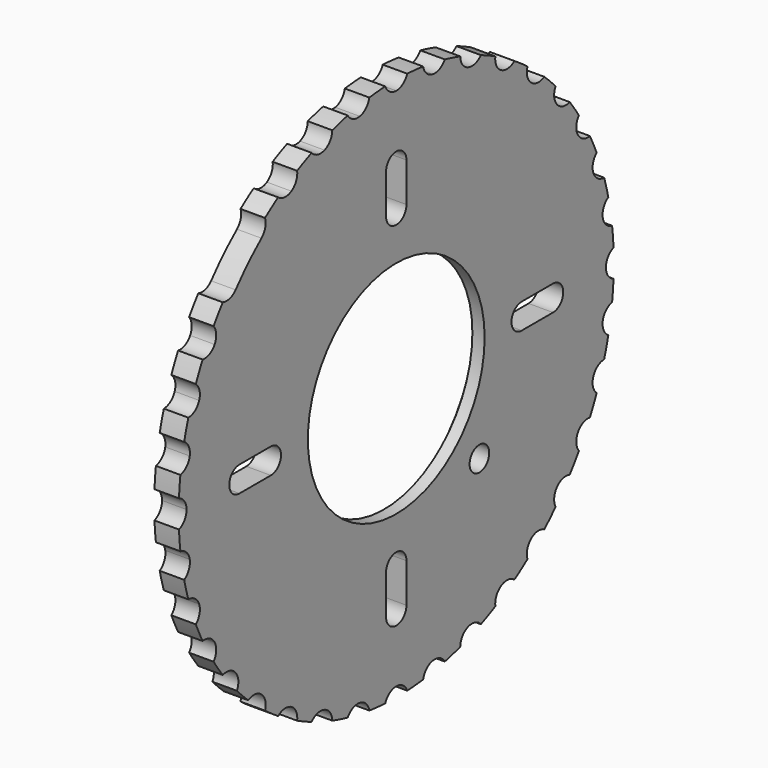
from build123d import *

# Parameters (mm, degrees)
F0_R     = 2.5
F0_R_2   = 26.25
F2_DEPTH = 5
F1_START = 2.5
F0_R_3   = 22.55
F1_DEPTH = 2.5


# Not quite as in the source:
# - a feature names something its author has since deleted; it is built from what else it names


with BuildPart() as f2:
    # F0 (on Right) → F2 (new body)
    with BuildSketch(Plane.YZ):
        with BuildLine():
            ThreePointArc((0, 53.5), (4.6628322594, 53.296416346), (9.2901775494, 52.6872147784))
            ThreePointArc((9.2901775494, 52.6872147784), (7.7067499567, 53.5035037785), (6.8653638665, 55.0737394679))
            ThreePointArc((6.8653638665, 55.0737394679), (4.8371437225, 55.2888057441), (2.8023909329, 55.4292035398))
            ThreePointArc((2.8023909329, 55.4292035398), (1.7011188406, 54.0289284328), (0, 53.5))
        make_face()
        with BuildLine():
            ThreePointArc((9.2901775494, 52.6872147784), (13.8468189413, 51.6770316989), (18.2980776808, 50.2735552073))
            ThreePointArc((18.2980776808, 50.2735552073), (16.8804530287, 51.3524022613), (16.3245180589, 53.0448876909))
            ThreePointArc((16.3245180589, 53.0448876909), (14.3644570032, 53.608883359), (12.3849965019, 54.1004793107))
            ThreePointArc((12.3849965019, 54.1004793107), (11.0573000071, 52.9127114302), (9.2901775494, 52.6872147784))
        make_face()
        with BuildLine():
            ThreePointArc((18.2980776808, 50.2735552073), (22.6100768811, 48.4874666634), (26.7499997548, 46.332359244))
            ThreePointArc((26.7499997548, 46.332359244), (25.5412520248, 47.6409841102), (25.2876600307, 49.4042938435))
            ThreePointArc((25.2876600307, 49.4042938435), (23.4553135266, 50.3000821805), (21.5912902193, 51.1279393939))
            ThreePointArc((21.5912902193, 51.1279393939), (20.0775106745, 50.1887684493), (18.2980776808, 50.2735552073))
        make_face()
        with BuildLine():
            ThreePointArc((26.7499997548, 46.332359244), (30.6863392453, 43.8246344391), (34.3891371491, 40.983377681))
            ThreePointArc((34.3891371491, 40.983377681), (33.4259931317, 42.4820184875), (33.4824492486, 44.2625755274))
            ThreePointArc((33.4824492486, 44.2625755274), (31.8334922175, 45.462938458), (30.1415435091, 46.6019029106))
            ThreePointArc((30.1415435091, 46.6019029106), (28.4876762061, 45.9398651305), (26.7499997548, 46.332359244))
        make_face()
        with BuildLine():
            ThreePointArc((34.3891371491, 40.983377681), (37.8302128361, 37.8302127508), (40.9833777585, 34.3891370567))
            ThreePointArc((40.9833777585, 34.3891370567), (40.2951022841, 36.0322583562), (40.659891189, 37.7759612518))
            ThreePointArc((40.659891189, 37.7759612518), (39.2444263559, 39.2444263559), (37.7759612518, 40.659891189))
            ThreePointArc((37.7759612518, 40.659891189), (36.0322584162, 40.2951022784), (34.3891371491, 40.983377681))
        make_face()
        with BuildLine():
            ThreePointArc((40.9833777585, 34.3891370567), (43.8246344309, 30.686339257), (46.3323591695, 26.7499998839))
            ThreePointArc((46.3323591695, 26.7499998839), (45.9398651365, 28.4876762804), (46.6019029106, 30.1415435091))
            ThreePointArc((46.6019029106, 30.1415435091), (45.462938458, 31.8334922175), (44.2625755274, 33.4824492486))
            ThreePointArc((44.2625755274, 33.4824492486), (42.4820185456, 33.4259931156), (40.9833777585, 34.3891370567))
        make_face()
        with BuildLine():
            ThreePointArc((46.3323591695, 26.7499998839), (48.4874666685, 22.6100768701), (50.2735552666, 18.298077518))
            ThreePointArc((50.2735552666, 18.298077518), (50.1887684276, 20.0775105907), (51.1279393939, 21.5912902193))
            ThreePointArc((51.1279393939, 21.5912902193), (50.3000821805, 23.4553135266), (49.4042938435, 25.2876600307))
            ThreePointArc((49.4042938435, 25.2876600307), (47.6409840429, 25.5412520568), (46.3323591695, 26.7499998839))
        make_face()
        with BuildLine():
            ThreePointArc((50.2735552666, 18.298077518), (51.6770317213, 13.8468188576), (52.6872147784, 9.2901775494))
            ThreePointArc((52.6872147784, 9.2901775494), (52.9127114302, 11.0573000071), (54.1004793107, 12.3849965019))
            ThreePointArc((54.1004793107, 12.3849965019), (53.608883359, 14.3644570032), (53.0448876909, 16.3245180589))
            ThreePointArc((53.0448876909, 16.3245180589), (51.3524023319, 16.8804529785), (50.2735552666, 18.298077518))
        make_face()
        with BuildLine():
            ThreePointArc((52.6872147784, 9.2901775494), (53.296416346, 4.6628322594), (53.5, 0))
            ThreePointArc((53.5, 0), (54.0289284328, 1.7011188406), (55.4292035398, 2.8023909329))
            ThreePointArc((55.4292035398, 2.8023909329), (55.2888057441, 4.8371437225), (55.0737394679, 6.8653638665))
            ThreePointArc((55.0737394679, 6.8653638665), (53.5035037785, 7.7067499567), (52.6872147784, 9.2901775494))
        make_face()
        with BuildLine():
            ThreePointArc((55.4292035398, -2.8023909329), (54.0289284328, -1.7011188406), (53.5, 0))
            ThreePointArc((53.5, 0), (53.2964163545, -4.6628321622), (52.6872148122, -9.2901773573))
            ThreePointArc((52.6872148122, -9.2901773573), (53.5035038469, -7.7067498872), (55.0737394679, -6.8653638665))
            ThreePointArc((55.0737394679, -6.8653638665), (55.2888057441, -4.8371437225), (55.4292035398, -2.8023909329))
        make_face()
        with BuildLine():
            ThreePointArc((54.1004793107, -12.3849965019), (52.9127113897, -11.0572999184), (52.6872148122, -9.2901773573))
            ThreePointArc((52.6872148122, -9.2901773573), (51.6770317241, -13.8468188471), (50.2735552073, -18.2980776808))
            ThreePointArc((50.2735552073, -18.2980776808), (51.3524022613, -16.8804530287), (53.0448876909, -16.3245180589))
            ThreePointArc((53.0448876909, -16.3245180589), (53.608883359, -14.3644570032), (54.1004793107, -12.3849965019))
        make_face()
        with BuildLine():
            ThreePointArc((51.1279393939, -21.5912902193), (50.1887684493, -20.0775106745), (50.2735552073, -18.2980776808))
            ThreePointArc((50.2735552073, -18.2980776808), (48.4874665555, -22.6100771125), (46.3323589886, -26.7500001972))
            ThreePointArc((46.3323589886, -26.7500001972), (47.6409838796, -25.5412521345), (49.4042938435, -25.2876600307))
            ThreePointArc((49.4042938435, -25.2876600307), (50.3000821805, -23.4553135266), (51.1279393939, -21.5912902193))
        make_face()
        with BuildLine():
            ThreePointArc((46.6019029106, -30.1415435091), (45.9398651508, -28.4876764607), (46.3323589886, -26.7500001972))
            ThreePointArc((46.3323589886, -26.7500001972), (43.8246342926, -30.6863394545), (40.983377681, -34.3891371491))
            ThreePointArc((40.983377681, -34.3891371491), (42.4820184875, -33.4259931317), (44.2625755274, -33.4824492486))
            ThreePointArc((44.2625755274, -33.4824492486), (45.462938458, -31.8334922175), (46.6019029106, -30.1415435091))
        make_face()
        with BuildLine():
            ThreePointArc((40.659891189, -37.7759612518), (40.2951022784, -36.0322584162), (40.983377681, -34.3891371491))
            ThreePointArc((40.983377681, -34.3891371491), (37.8302127508, -37.8302128361), (34.3891370567, -40.9833777585))
            ThreePointArc((34.3891370567, -40.9833777585), (36.0322583562, -40.2951022841), (37.7759612518, -40.659891189))
            ThreePointArc((37.7759612518, -40.659891189), (39.2444263559, -39.2444263559), (40.659891189, -37.7759612518))
        make_face()
        with BuildLine():
            ThreePointArc((33.4824492486, -44.2625755274), (33.4259931156, -42.4820185456), (34.3891370567, -40.9833777585))
            ThreePointArc((34.3891370567, -40.9833777585), (30.6863393252, -43.8246343832), (26.7500000282, -46.3323590862))
            ThreePointArc((26.7500000282, -46.3323590862), (28.4876763634, -45.9398651431), (30.1415435091, -46.6019029106))
            ThreePointArc((30.1415435091, -46.6019029106), (31.8334922175, -45.462938458), (33.4824492486, -44.2625755274))
        make_face()
        with BuildLine():
            ThreePointArc((25.2876600307, -49.4042938435), (25.5412520926, -47.6409839676), (26.7500000282, -46.3323590862))
            ThreePointArc((26.7500000282, -46.3323590862), (22.6100771125, -48.4874665555), (18.298077864, -50.2735551407))
            ThreePointArc((18.298077864, -50.2735551407), (20.0775107689, -50.1887684738), (21.5912902193, -51.1279393939))
            ThreePointArc((21.5912902193, -51.1279393939), (23.4553135266, -50.3000821805), (25.2876600307, -49.4042938435))
        make_face()
        with BuildLine():
            ThreePointArc((16.3245180589, -53.0448876909), (16.8804530853, -51.3524021819), (18.298077864, -50.2735551407))
            ThreePointArc((18.298077864, -50.2735551407), (13.8468189413, -51.6770316989), (9.2901773573, -52.6872148122))
            ThreePointArc((9.2901773573, -52.6872148122), (11.0572999184, -52.9127113897), (12.3849965019, -54.1004793107))
            ThreePointArc((12.3849965019, -54.1004793107), (14.3644570032, -53.608883359), (16.3245180589, -53.0448876909))
        make_face()
        with BuildLine():
            ThreePointArc((6.8653638665, -55.0737394679), (7.7067498872, -53.5035038469), (9.2901773573, -52.6872148122))
            ThreePointArc((9.2901773573, -52.6872148122), (4.6628321622, -53.2964163544), (0, -53.5))
            ThreePointArc((0, -53.5), (1.7011188406, -54.0289284328), (2.8023909329, -55.4292035398))
            ThreePointArc((2.8023909329, -55.4292035398), (4.8371437225, -55.2888057441), (6.8653638665, -55.0737394679))
        make_face()
        with BuildLine():
            ThreePointArc((-2.8023909329, -55.4292035398), (-1.7011188406, -54.0289284328), (0, -53.5))
            ThreePointArc((0, -53.5), (-4.6628322344, -53.2964163481), (-9.2901775, -52.6872147871))
            ThreePointArc((-9.2901775, -52.6872147871), (-7.7067499388, -53.5035037961), (-6.8653638665, -55.0737394679))
            ThreePointArc((-6.8653638665, -55.0737394679), (-4.8371437225, -55.2888057441), (-2.8023909329, -55.4292035398))
        make_face()
        with BuildLine():
            ThreePointArc((-12.3849965019, -54.1004793107), (-11.0572999842, -52.9127114198), (-9.2901775, -52.6872147871))
            ThreePointArc((-9.2901775, -52.6872147871), (-13.8468189171, -51.6770317054), (-18.2980776808, -50.2735552073))
            ThreePointArc((-18.2980776808, -50.2735552073), (-16.8804530287, -51.3524022613), (-16.3245180589, -53.0448876909))
            ThreePointArc((-16.3245180589, -53.0448876909), (-14.3644570032, -53.608883359), (-12.3849965019, -54.1004793107))
        make_face()
        with BuildLine():
            ThreePointArc((-21.5912902193, -51.1279393939), (-20.0775106745, -50.1887684493), (-18.2980776808, -50.2735552073))
            ThreePointArc((-18.2980776808, -50.2735552073), (-22.6100770517, -48.4874665838), (-26.7500000809, -46.3323590558))
            ThreePointArc((-26.7500000809, -46.3323590558), (-25.5412521057, -47.6409839402), (-25.2876600307, -49.4042938435))
            ThreePointArc((-25.2876600307, -49.4042938435), (-23.4553135266, -50.3000821805), (-21.5912902193, -51.1279393939))
        make_face()
        with BuildLine():
            ThreePointArc((-30.1415435091, -46.6019029106), (-28.4876763937, -45.9398651455), (-26.7500000809, -46.3323590558))
            ThreePointArc((-26.7500000809, -46.3323590558), (-30.6863394301, -43.8246343097), (-34.3891372062, -40.983377633))
            ThreePointArc((-34.3891372062, -40.983377633), (-33.4259931416, -42.4820184516), (-33.4824492486, -44.2625755274))
            ThreePointArc((-33.4824492486, -44.2625755274), (-31.8334922175, -45.462938458), (-30.1415435091, -46.6019029106))
        make_face()
        with BuildLine():
            ThreePointArc((-37.7759612518, -40.659891189), (-36.0322584533, -40.2951022748), (-34.3891372062, -40.983377633))
            ThreePointArc((-34.3891372062, -40.983377633), (-37.8302128361, -37.8302127508), (-40.9833777106, -34.3891371138))
            ThreePointArc((-40.9833777106, -34.3891371138), (-40.2951022806, -36.0322583933), (-40.659891189, -37.7759612518))
            ThreePointArc((-40.659891189, -37.7759612518), (-39.2444263559, -39.2444263559), (-37.7759612518, -40.659891189))
        make_face()
        with BuildLine():
            ThreePointArc((-44.2625755274, -33.4824492486), (-42.4820185097, -33.4259931256), (-40.9833777106, -34.3891371138))
            ThreePointArc((-40.9833777106, -34.3891371138), (-43.8246343882, -30.686339318), (-46.3323591322, -26.7499999484))
            ThreePointArc((-46.3323591322, -26.7499999484), (-45.9398651394, -28.4876763175), (-46.6019029106, -30.1415435091))
            ThreePointArc((-46.6019029106, -30.1415435091), (-45.462938458, -31.8334922175), (-44.2625755274, -33.4824492486))
        make_face()
        with BuildLine():
            ThreePointArc((-49.4042938435, -25.2876600307), (-47.6409840092, -25.5412520728), (-46.3323591322, -26.7499999484))
            ThreePointArc((-46.3323591322, -26.7499999484), (-48.4874666416, -22.6100769278), (-50.2735552486, -18.2980775676))
            ThreePointArc((-50.2735552486, -18.2980775676), (-50.1887684342, -20.0775106162), (-51.1279393939, -21.5912902193))
            ThreePointArc((-51.1279393939, -21.5912902193), (-50.3000821805, -23.4553135266), (-49.4042938435, -25.2876600307))
        make_face()
        with BuildLine():
            ThreePointArc((-53.0448876909, -16.3245180589), (-51.3524023104, -16.8804529938), (-50.2735552486, -18.2980775676))
            ThreePointArc((-50.2735552486, -18.2980775676), (-51.6770317301, -13.8468188249), (-52.6872147993, -9.2901774307))
            ThreePointArc((-52.6872147993, -9.2901774307), (-52.9127114052, -11.0572999522), (-54.1004793107, -12.3849965019))
            ThreePointArc((-54.1004793107, -12.3849965019), (-53.608883359, -14.3644570032), (-53.0448876909, -16.3245180589))
        make_face()
        with BuildLine():
            ThreePointArc((-55.0737394679, -6.8653638665), (-53.5035038207, -7.7067499137), (-52.6872147993, -9.2901774307))
            ThreePointArc((-52.6872147993, -9.2901774307), (-53.2964163512, -4.6628321993), (-53.5, 0))
            ThreePointArc((-53.5, 0), (-54.0289284328, -1.7011188406), (-55.4292035398, -2.8023909329))
            ThreePointArc((-55.4292035398, -2.8023909329), (-55.2888057441, -4.8371437225), (-55.0737394679, -6.8653638665))
        make_face()
        with BuildLine():
            ThreePointArc((-53.5, 0), (-53.296416346, 4.6628322594), (-52.6872147784, 9.2901775494))
            ThreePointArc((-52.6872147784, 9.2901775494), (-53.5035037785, 7.7067499567), (-55.0737394679, 6.8653638665))
            ThreePointArc((-55.0737394679, 6.8653638665), (-55.2888057441, 4.8371437225), (-55.4292035398, 2.8023909329))
            ThreePointArc((-55.4292035398, 2.8023909329), (-54.0289284328, 1.7011188406), (-53.5, 0))
        make_face()
        with BuildLine():
            ThreePointArc((-52.6872147784, 9.2901775494), (-51.6770316989, 13.8468189413), (-50.2735552073, 18.2980776808))
            ThreePointArc((-50.2735552073, 18.2980776808), (-51.3524022613, 16.8804530287), (-53.0448876909, 16.3245180589))
            ThreePointArc((-53.0448876909, 16.3245180589), (-53.608883359, 14.3644570032), (-54.1004793107, 12.3849965019))
            ThreePointArc((-54.1004793107, 12.3849965019), (-52.9127114302, 11.0573000071), (-52.6872147784, 9.2901775494))
        make_face()
        with BuildLine():
            ThreePointArc((-50.2735552073, 18.2980776808), (-48.4874665965, 22.6100770244), (-46.3323590859, 26.7500000287))
            ThreePointArc((-46.3323590859, 26.7500000287), (-47.6409839674, 25.5412520927), (-49.4042938435, 25.2876600307))
            ThreePointArc((-49.4042938435, 25.2876600307), (-50.3000821805, 23.4553135266), (-51.1279393939, 21.5912902193))
            ThreePointArc((-51.1279393939, 21.5912902193), (-50.1887684493, 20.0775106745), (-50.2735552073, 18.2980776808))
        make_face()
        with BuildLine():
            ThreePointArc((-46.3323590859, 26.7500000287), (-43.8246343484, 30.6863393749), (-40.983377681, 34.3891371491))
            ThreePointArc((-40.983377681, 34.3891371491), (-42.4820184875, 33.4259931317), (-44.2625755274, 33.4824492486))
            ThreePointArc((-44.2625755274, 33.4824492486), (-45.462938458, 31.8334922175), (-46.6019029106, 30.1415435091))
            ThreePointArc((-46.6019029106, 30.1415435091), (-45.9398651431, 28.4876763637), (-46.3323590859, 26.7500000287))
        make_face()
        with BuildLine():
            ThreePointArc((-34.3891371491, 40.983377681), (-30.6863393263, 43.8246343824), (-26.749999926, 46.3323591452))
            ThreePointArc((-26.749999926, 46.3323591452), (-28.4876763046, 45.9398651384), (-30.1415435091, 46.6019029106))
            ThreePointArc((-30.1415435091, 46.6019029106), (-31.8334922175, 45.462938458), (-33.4824492486, 44.2625755274))
            ThreePointArc((-33.4824492486, 44.2625755274), (-33.4259931317, 42.4820184875), (-34.3891371491, 40.983377681))
        make_face()
        with BuildLine():
            ThreePointArc((-26.749999926, 46.3323591452), (-22.6100769706, 48.4874666216), (-18.2980776808, 50.2735552073))
            ThreePointArc((-18.2980776808, 50.2735552073), (-20.0775106745, 50.1887684493), (-21.5912902193, 51.1279393939))
            ThreePointArc((-21.5912902193, 51.1279393939), (-23.4553135266, 50.3000821805), (-25.2876600307, 49.4042938435))
            ThreePointArc((-25.2876600307, 49.4042938435), (-25.5412520672, 47.6409840209), (-26.749999926, 46.3323591452))
        make_face()
        with BuildLine():
            ThreePointArc((52.6872148122, -9.2901773573), (53.2964163545, -4.6628321622), (53.5, 0))
            ThreePointArc((53.5, 0), (53.296416346, 4.6628322594), (52.6872147784, 9.2901775494))
            ThreePointArc((52.6872147784, 9.2901775494), (51.6770317213, 13.8468188576), (50.2735552666, 18.298077518))
            ThreePointArc((50.2735552666, 18.298077518), (48.4874666685, 22.6100768701), (46.3323591695, 26.7499998839))
            ThreePointArc((46.3323591695, 26.7499998839), (43.8246344309, 30.686339257), (40.9833777585, 34.3891370567))
            ThreePointArc((40.9833777585, 34.3891370567), (37.8302128361, 37.8302127508), (34.3891371491, 40.983377681))
            ThreePointArc((34.3891371491, 40.983377681), (30.6863392453, 43.8246344391), (26.7499997548, 46.332359244))
            ThreePointArc((26.7499997548, 46.332359244), (22.6100768811, 48.4874666634), (18.2980776808, 50.2735552073))
            ThreePointArc((18.2980776808, 50.2735552073), (13.8468189413, 51.6770316989), (9.2901775494, 52.6872147784))
            ThreePointArc((9.2901775494, 52.6872147784), (4.6628322594, 53.296416346), (0, 53.5))
            ThreePointArc((0, 53.5), (-4.6628322594, 53.296416346), (-9.2901775494, 52.6872147784))
            ThreePointArc((-9.2901775494, 52.6872147784), (-13.8468189413, 51.6770316989), (-18.2980776808, 50.2735552073))
            ThreePointArc((-18.2980776808, 50.2735552073), (-22.6100769706, 48.4874666216), (-26.749999926, 46.3323591452))
            ThreePointArc((-26.749999926, 46.3323591452), (-30.6863393263, 43.8246343824), (-34.3891371491, 40.983377681))
            ThreePointArc((-34.3891371491, 40.983377681), (-37.8302127935, 37.8302127935), (-40.983377681, 34.3891371491))
            ThreePointArc((-40.983377681, 34.3891371491), (-43.8246343484, 30.6863393749), (-46.3323590859, 26.7500000287))
            ThreePointArc((-46.3323590859, 26.7500000287), (-48.4874665965, 22.6100770244), (-50.2735552073, 18.2980776808))
            ThreePointArc((-50.2735552073, 18.2980776808), (-51.6770316989, 13.8468189413), (-52.6872147784, 9.2901775494))
            ThreePointArc((-52.6872147784, 9.2901775494), (-53.296416346, 4.6628322594), (-53.5, 0))
            ThreePointArc((-53.5, 0), (-53.2964163512, -4.6628321993), (-52.6872147993, -9.2901774307))
            ThreePointArc((-52.6872147993, -9.2901774307), (-51.6770317301, -13.8468188249), (-50.2735552486, -18.2980775676))
            ThreePointArc((-50.2735552486, -18.2980775676), (-48.4874666416, -22.6100769278), (-46.3323591322, -26.7499999484))
            ThreePointArc((-46.3323591322, -26.7499999484), (-43.8246343882, -30.686339318), (-40.9833777106, -34.3891371138))
            ThreePointArc((-40.9833777106, -34.3891371138), (-37.8302128361, -37.8302127508), (-34.3891372062, -40.983377633))
            ThreePointArc((-34.3891372062, -40.983377633), (-30.6863394301, -43.8246343097), (-26.7500000809, -46.3323590558))
            ThreePointArc((-26.7500000809, -46.3323590558), (-22.6100770517, -48.4874665838), (-18.2980776808, -50.2735552073))
            ThreePointArc((-18.2980776808, -50.2735552073), (-13.8468189171, -51.6770317054), (-9.2901775, -52.6872147871))
            ThreePointArc((-9.2901775, -52.6872147871), (-4.6628322344, -53.2964163481), (0, -53.5))
            ThreePointArc((0, -53.5), (4.6628321622, -53.2964163544), (9.2901773573, -52.6872148122))
            ThreePointArc((9.2901773573, -52.6872148122), (13.8468189413, -51.6770316989), (18.298077864, -50.2735551407))
            ThreePointArc((18.298077864, -50.2735551407), (22.6100771125, -48.4874665555), (26.7500000282, -46.3323590862))
            ThreePointArc((26.7500000282, -46.3323590862), (30.6863393252, -43.8246343832), (34.3891370567, -40.9833777585))
            ThreePointArc((34.3891370567, -40.9833777585), (37.8302127508, -37.8302128361), (40.983377681, -34.3891371491))
            ThreePointArc((40.983377681, -34.3891371491), (43.8246342926, -30.6863394545), (46.3323589886, -26.7500001972))
            ThreePointArc((46.3323589886, -26.7500001972), (48.4874665555, -22.6100771125), (50.2735552073, -18.2980776808))
            ThreePointArc((50.2735552073, -18.2980776808), (51.6770317241, -13.8468188471), (52.6872148122, -9.2901773573))
        make_face()
        with BuildLine():
            Line((-2.6, -40), (-2.6, -32))
            ThreePointArc((-2.6, -32), (0, -29.4), (2.6, -32))
            Line((2.6, -32), (2.6, -40))
            ThreePointArc((2.6, -40), (0, -42.6), (-2.6, -40))
        make_face(mode=Mode.SUBTRACT)
        with Locations((21.2132034356, -21.2132034356)):
            Circle(F0_R, mode=Mode.SUBTRACT)
        with BuildLine():
            Line((-40, 2.6), (-32, 2.6))
            ThreePointArc((-32, 2.6), (-29.4, 0), (-32, -2.6))
            Line((-32, -2.6), (-40, -2.6))
            ThreePointArc((-40, -2.6), (-42.6, 0), (-40, 2.6))
        make_face(mode=Mode.SUBTRACT)
        Circle(F0_R_2, mode=Mode.SUBTRACT)
        with BuildLine():
            Line((40, -2.6), (32, -2.6))
            ThreePointArc((32, -2.6), (29.4, 0), (32, 2.6))
            Line((32, 2.6), (40, 2.6))
            ThreePointArc((40, 2.6), (42.6, 0), (40, -2.6))
        make_face(mode=Mode.SUBTRACT)
        with BuildLine():
            Line((-2.6, 32), (-2.6, 40))
            ThreePointArc((-2.6, 40), (0, 42.6), (2.6, 40))
            Line((2.6, 40), (2.6, 32))
            ThreePointArc((2.6, 32), (0, 29.4), (-2.6, 32))
        make_face(mode=Mode.SUBTRACT)
        with BuildLine():
            ThreePointArc((-18.2980776808, 50.2735552073), (-13.8468189413, 51.6770316989), (-9.2901775494, 52.6872147784))
            ThreePointArc((-9.2901775494, 52.6872147784), (-11.0573000071, 52.9127114302), (-12.3849965019, 54.1004793107))
            ThreePointArc((-12.3849965019, 54.1004793107), (-14.3644570032, 53.608883359), (-16.3245180589, 53.0448876909))
            ThreePointArc((-16.3245180589, 53.0448876909), (-16.8804530287, 51.3524022613), (-18.2980776808, 50.2735552073))
        make_face()
        with BuildLine():
            ThreePointArc((-9.2901775494, 52.6872147784), (-4.6628322594, 53.296416346), (0, 53.5))
            ThreePointArc((0, 53.5), (-1.7011188406, 54.0289284328), (-2.8023909329, 55.4292035398))
            ThreePointArc((-2.8023909329, 55.4292035398), (-4.8371437225, 55.2888057441), (-6.8653638665, 55.0737394679))
            ThreePointArc((-6.8653638665, 55.0737394679), (-7.7067499567, 53.5035037785), (-9.2901775494, 52.6872147784))
        make_face()
    extrude(amount=F2_DEPTH)

    # F0 (on Right) → F1 (join)
    with BuildSketch(Plane.YZ.offset(F1_START)):
        Circle(F0_R_2)
        Circle(F0_R_3, mode=Mode.SUBTRACT)
    extrude(amount=F1_DEPTH)


solid = f2.part
